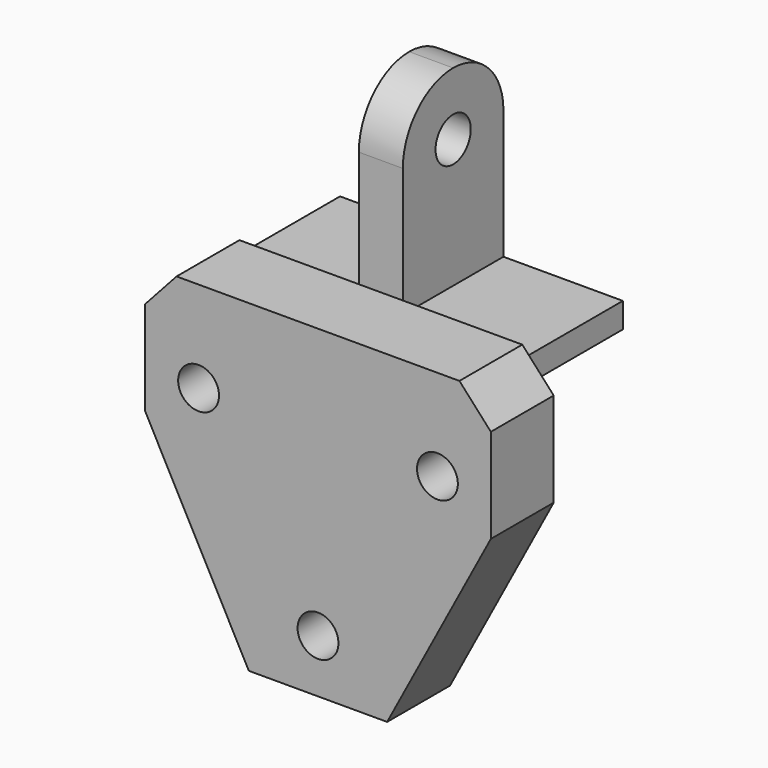
from build123d import *

# Parameters (mm, degrees)
F0_R     = 6.5
F1_DEPTH = 25
F3_DEPTH = 40
F4_R     = 19.99999
F5_R     = 7
F6_DEPTH = 25


# Not quite as in the source:
# - a fillet or chamfer is up to 0.001 mm smaller than in the source, because OpenCascade refuses the exact size


with BuildPart() as f1:
    # F0 (on Front) → F1 (new body)
    with BuildSketch(Plane.XZ):
        with BuildLine():
            Line((0, -28.0120762104), (0, 51.4879237896))
            Line((0, 51.4879237896), (-45, 51.4879237896))
            Line((-45, 51.4879237896), (-55, 40.4879237896))
            Line((-55, 40.4879237896), (-55, 10.4879237896))
            Line((-55, 10.4879237896), (-22, -51.5120762104))
            Line((-22, -51.5120762104), (0, -51.5120762104))
            Line((0, -51.5120762104), (0, -41.0120762104))
            ThreePointArc((0, -41.0120762104), (-6.5, -34.5120762104), (0, -28.0120762104))
        make_face()
        with Locations((-38, 22.4879237896)):
            Circle(F0_R, mode=Mode.SUBTRACT)
        with BuildLine():
            Line((45, 51.4879237896), (0, 51.4879237896))
            Line((0, 51.4879237896), (0, -28.0120762104))
            ThreePointArc((0, -28.0120762104), (6.5, -34.5120762104), (0, -41.0120762104))
            Line((0, -41.0120762104), (0, -51.5120762104))
            Line((0, -51.5120762104), (22, -51.5120762104))
            Line((22, -51.5120762104), (55, 10.4879237896))
            Line((55, 10.4879237896), (55, 40.4879237896))
            Line((55, 40.4879237896), (45, 51.4879237896))
        make_face()
        with Locations((38, 22.4879237896)):
            Circle(F0_R, mode=Mode.SUBTRACT)
    extrude(amount=F1_DEPTH)

    # F2 (on face) → F3 (join)
    with BuildSketch(Plane(origin=(0, 0, 0), x_dir=(-1, 0, 0), z_dir=(0, 1, 0))):
        Polygon((7, 108.4879237896), (0, 108.4879237896), (-7, 108.4879237896), (-7, 47.4879237896), (-45, 47.4879237896), (-45, 39.4879237896), (-7, 39.4879237896), (-7, -14.5120762104), (0, -14.5120762104), (7, -14.5120762104), (7, 39.4879237896), (45, 39.4879237896), (45, 47.4879237896), (7, 47.4879237896), align=None)
    extrude(amount=F3_DEPTH)

    # F4 (radius 20 in the source; OpenCascade refuses exactly that, so slightly less here)
    f4_edges = [f1.edges().sort_by_distance(p)[0] for p in [
        (0, 0, 108.487924),
        (0, 40, 108.487924),
    ]]
    fillet(f4_edges, radius=F4_R)

    # F5 (on face) → F6 (cut)
    with BuildSketch(Plane.YZ.offset(7)):
        with Locations((20, 88.4879237896)):
            Circle(F5_R)
        Polygon((40, -14.5120762104), (40, 24.4879237896), (17, -14.5120762104), align=None)
    extrude(amount=-F6_DEPTH, mode=Mode.SUBTRACT)


solid = f1.part
